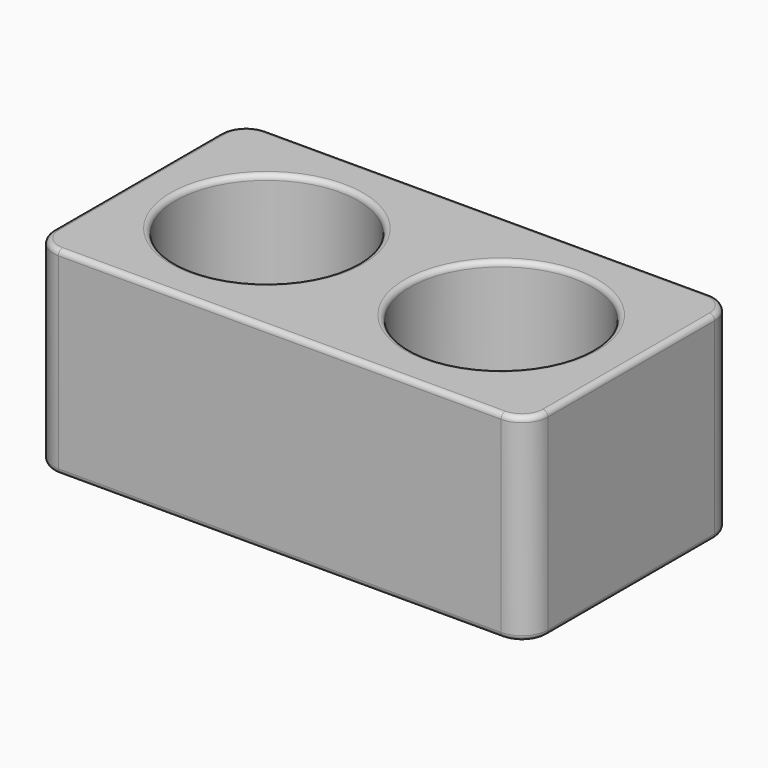
from build123d import *

# Parameters (mm, degrees)
F0_W         = 95
F0_H         = 50
F0_R         = 17.5
F1_DEPTH     = 36
F2_W         = 95
F2_H         = 50
F3_DEPTH     = 2
F4_R         = 1
F5_T1_DEPTH  = 38
F5_T4_ANGLE  = 90
F5_T6_ANGLE  = 90
F5_T8_ANGLE  = 90
F5_T10_ANGLE = 90
F5_T12_ANGLE = 90
F5_T14_ANGLE = 90
F5_T16_ANGLE = 90
F5_T18_ANGLE = 90


# Not quite as in the source:
# - a fillet or chamfer that OpenCascade refuses, or shapes differently, is made with other operations: its cross-section is extruded or revolved along the edge and cut away or added


with BuildPart() as f1:
    # F0 (on Top) → F1 (new body)
    with BuildSketch(Plane.XY):
        Rectangle(F0_W, F0_H)
        with Locations((-22.5, 0)):
            Circle(F0_R, mode=Mode.SUBTRACT)
        with Locations((22.5, 0)):
            Circle(F0_R, mode=Mode.SUBTRACT)
    extrude(amount=F1_DEPTH)

    # F2 (on face) → F3 (join)
    with BuildSketch(Plane(origin=(0, 0, 0), x_dir=(1, 0, 0), z_dir=(0, 0, -1))):
        Rectangle(F2_W, F2_H)
    extrude(amount=F3_DEPTH)

    # F4
    f4_edges = [f1.edges().sort_by_distance(p)[0] for p in [
        (0, 25, 36),
        (-47.5, 0, 36),
        (0, -25, 36),
        (47.5, 0, 36),
        (-40, 0, 36),
        (5, 0, 36),
        (0, 25, -2),
        (47.5, 0, -2),
        (0, -25, -2),
        (-47.5, 0, -2),
    ]]
    fillet(f4_edges, radius=F4_R)

    # F5: fillet of radius 5 on 4 edges, made by hand

    # F5_s2 → F5_t1 (cut)
    with BuildSketch(Plane.XY.offset(-2)):
        with BuildLine():
            ThreePointArc((42.5, 25), (46.0355339059, 23.5355339059), (47.5, 20))
            Line((47.5, 20), (47.5, 25))
            Line((47.5, 25), (42.5, 25))
        make_face()
        with BuildLine():
            ThreePointArc((47.5, -20), (46.0355339059, -23.5355339059), (42.5, -25))
            Line((42.5, -25), (47.5, -25))
            Line((47.5, -25), (47.5, -20))
        make_face()
        with BuildLine():
            ThreePointArc((-47.5, -20), (-46.0355339059, -23.5355339059), (-42.5, -25))
            Line((-42.5, -25), (-47.5, -25))
            Line((-47.5, -25), (-47.5, -20))
        make_face()
        with BuildLine():
            ThreePointArc((-42.5, 25), (-46.0355339059, 23.5355339059), (-47.5, 20))
            Line((-47.5, 20), (-47.5, 25))
            Line((-47.5, 25), (-42.5, 25))
        make_face()
    extrude(amount=F5_T1_DEPTH, mode=Mode.SUBTRACT)

    # F5_s3 → F5_t4 (revolve, cut)
    with BuildSketch(Plane.XZ.offset(-20)):
        with BuildLine():
            ThreePointArc((-46.5, -2), (-47.2071067812, -1.7071067812), (-47.5, -1))
            Line((-47.5, -1), (-47.5, -2))
            Line((-47.5, -2), (-46.5, -2))
        make_face()
    revolve(axis=Axis((-42.5, 20, -2), (0, 0, -1)), revolution_arc=F5_T4_ANGLE, mode=Mode.SUBTRACT)

    # F5_s5 → F5_t6 (revolve, cut)
    with BuildSketch(Plane.YZ.offset(-42.5)):
        with BuildLine():
            ThreePointArc((24, 36), (24.7071067812, 35.7071067812), (25, 35))
            Line((25, 35), (25, 36))
            Line((25, 36), (24, 36))
        make_face()
    revolve(axis=Axis((-42.5, 20, 36), (0, 0, 1)), revolution_arc=F5_T6_ANGLE, mode=Mode.SUBTRACT)

    # F5_s7 → F5_t8 (revolve, cut)
    with BuildSketch(Plane.YZ.offset(-42.5)):
        with BuildLine():
            ThreePointArc((-24, -2), (-24.7071067812, -1.7071067812), (-25, -1))
            Line((-25, -1), (-25, -2))
            Line((-25, -2), (-24, -2))
        make_face()
    revolve(axis=Axis((-42.5, -20, -2), (0, 0, -1)), revolution_arc=F5_T8_ANGLE, mode=Mode.SUBTRACT)

    # F5_s9 → F5_t10 (revolve, cut)
    with BuildSketch(Plane.XZ.offset(20)):
        with BuildLine():
            ThreePointArc((-46.5, 36), (-47.2071067812, 35.7071067812), (-47.5, 35))
            Line((-47.5, 35), (-47.5, 36))
            Line((-47.5, 36), (-46.5, 36))
        make_face()
    revolve(axis=Axis((-42.5, -20, 36), (0, 0, 1)), revolution_arc=F5_T10_ANGLE, mode=Mode.SUBTRACT)

    # F5_s11 → F5_t12 (revolve, cut)
    with BuildSketch(Plane.YZ.offset(42.5)):
        with BuildLine():
            ThreePointArc((-24, 36), (-24.7071067812, 35.7071067812), (-25, 35))
            Line((-25, 35), (-25, 36))
            Line((-25, 36), (-24, 36))
        make_face()
    revolve(axis=Axis((42.5, -20, 36), (0, 0, 1)), revolution_arc=F5_T12_ANGLE, mode=Mode.SUBTRACT)

    # F5_s13 → F5_t14 (revolve, cut)
    with BuildSketch(Plane.XZ.offset(20)):
        with BuildLine():
            ThreePointArc((46.5, -2), (47.2071067812, -1.7071067812), (47.5, -1))
            Line((47.5, -1), (47.5, -2))
            Line((47.5, -2), (46.5, -2))
        make_face()
    revolve(axis=Axis((42.5, -20, -2), (0, 0, -1)), revolution_arc=F5_T14_ANGLE, mode=Mode.SUBTRACT)

    # F5_s15 → F5_t16 (revolve, cut)
    with BuildSketch(Plane.XZ.offset(-20)):
        with BuildLine():
            ThreePointArc((46.5, 36), (47.2071067812, 35.7071067812), (47.5, 35))
            Line((47.5, 35), (47.5, 36))
            Line((47.5, 36), (46.5, 36))
        make_face()
    revolve(axis=Axis((42.5, 20, 36), (0, 0, 1)), revolution_arc=F5_T16_ANGLE, mode=Mode.SUBTRACT)

    # F5_s17 → F5_t18 (revolve, cut)
    with BuildSketch(Plane.YZ.offset(42.5)):
        with BuildLine():
            ThreePointArc((24, -2), (24.7071067812, -1.7071067812), (25, -1))
            Line((25, -1), (25, -2))
            Line((25, -2), (24, -2))
        make_face()
    revolve(axis=Axis((42.5, 20, -2), (0, 0, -1)), revolution_arc=F5_T18_ANGLE, mode=Mode.SUBTRACT)


solid = f1.part
